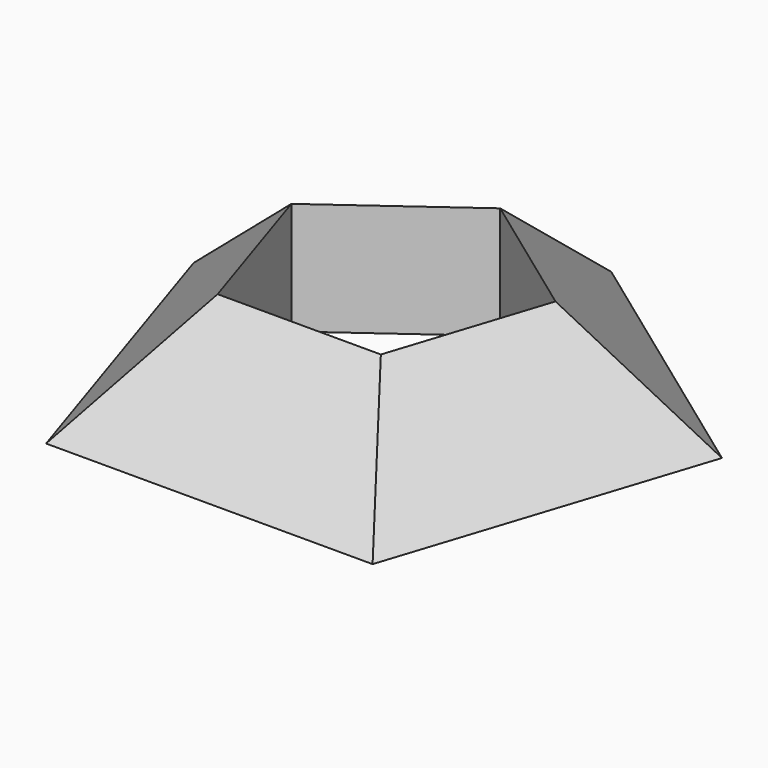
from build123d import *

# Parameters (mm, degrees)
F1_DEPTH = 30
F1_TAPER = 45
F3_DEPTH = 30


with BuildPart() as f1:
    # F0 (on Top) → F1 (new body)
    with BuildSketch(Plane.XY):
        Polygon((0, 74.164079), (-70.53423, 22.917961), (-43.592552, -60), (43.592552, -60), (70.53423, 22.917961), align=None)
    extrude(amount=F1_DEPTH, taper=F1_TAPER)

    # F3 (cut): a face of the model
    f3_faces = [f1.faces().sort_by_distance(p)[0] for p in [
        (0, 0, 30),
    ]]
    extrude(f3_faces, amount=-F3_DEPTH, mode=Mode.SUBTRACT)


solid = f1.part
